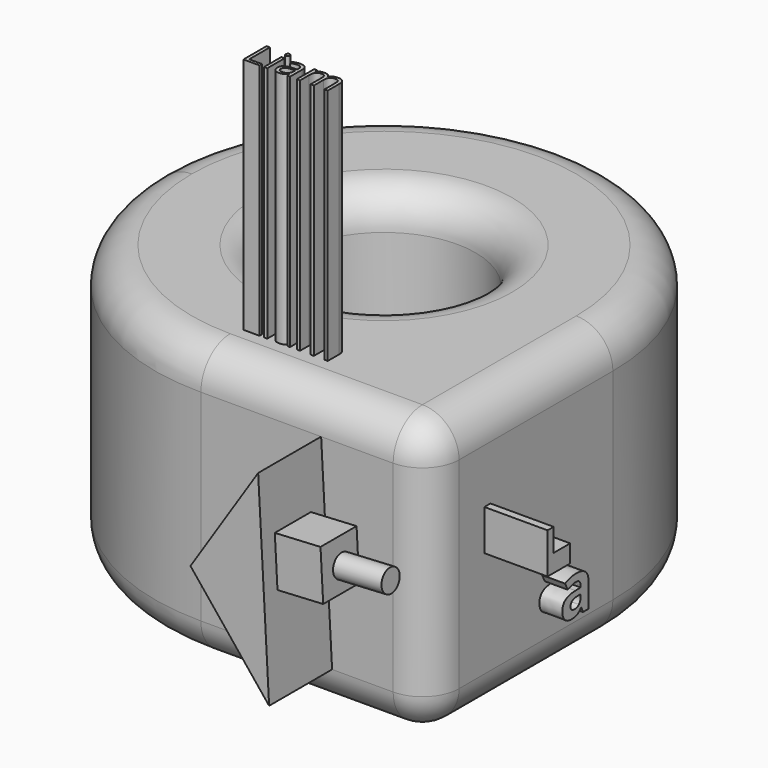
from build123d import *

# Parameters (mm, degrees)
F0_W          = 127
F0_H          = 127
F1_DEPTH      = 76.2
F3_DEPTH      = 84.582
F4_R          = 63.49999
F5_R          = 25.4
F6_DEPTH      = 85.09
F7_R          = 10.16
F9_DEPTH      = 21.844
F10_W         = 12.5058554592
F10_H         = 13.7337893248
F11_DEPTH     = 12.7
F12_R         = 3.150764017
F13_DEPTH     = 13.462
F15_DEPTH     = 17.526
F17_DEPTH     = 6.35
F18_TEXT_SIZE = 11.2532431053
F19_DEPTH     = 66.04


# Not quite as in the source:
# - a fillet or chamfer is up to 0.001 mm smaller than in the source, because OpenCascade refuses the exact size
# - Text() gives the source's letters only with a copy of the font that has no kerning and outlines rounded to 1/6400 em; it was checked with that copy


with BuildPart() as f1:
    # F0 (on Top) → F1 (new body)
    with BuildSketch(Plane.XY):
        Rectangle(F0_W, F0_H)
    extrude(amount=F1_DEPTH)

    # F2 (on face) → F3 (cut)
    with BuildSketch(Plane.XY.offset(76.2)):
        with BuildLine():
            ThreePointArc((1.088e-07, 63.5), (44.9012806438, 44.9012805669), (63.5, 0))
            Line((63.5, 0), (63.5, 63.5))
            Line((63.5, 63.5), (1.088e-07, 63.5))
        make_face()
        with BuildLine():
            ThreePointArc((-63.5, 0), (-44.9012805669, 44.9012806438), (1.088e-07, 63.5))
            Line((1.088e-07, 63.5), (-63.5, 63.5))
            Line((-63.5, 63.5), (-63.5, 0))
        make_face()
    extrude(amount=-F3_DEPTH, mode=Mode.SUBTRACT)

    # F4 (radius 63.5 in the source; OpenCascade refuses exactly that, so slightly less here)
    f4_edges = [f1.edges().sort_by_distance(p)[0] for p in [
        (-63.5, -63.5, 38.1),
    ]]
    fillet(f4_edges, radius=F4_R)

    # F5 (on face) → F6 (cut)
    with BuildSketch(Plane.XY.offset(76.2)):
        Circle(F5_R)
    extrude(amount=-F6_DEPTH, mode=Mode.SUBTRACT)

    # F7
    f7_edges = [f1.edges().sort_by_distance(p)[0] for p in [
        (63.5, -31.75, 0),
        (63.5, 0, 38.1),
        (63.5, -31.75, 76.2),
        (63.5, -63.5, 38.1),
        (31.749995, -63.5, 0),
        (-1e-05, -63.5, 38.1),
        (31.749995, -63.5, 76.2),
        (-25.4, 0, 76.2),
        (25.4, 0, 38.1),
        (-25.4, 0, 0),
    ]]
    fillet(f7_edges, radius=F7_R)

    # F8 (on face) → F9 (join)
    with BuildSketch(Plane.XZ.offset(63.5)):
        Polygon((33.3577431738, 66.04), (14.5826684311, 37.2163690627), (36.4012047648, 10.16), align=None)
    extrude(amount=F9_DEPTH)

    # F10 (on face) → F11 (join)
    with BuildSketch(Plane(origin=(36.8452653483, 0, 2.0067492824), x_dir=(0, 1, 0), z_dir=(0.998520115, 0, 0.0543836367))):
        with Locations((-74.422, 41.0005301237)):
            Rectangle(F10_W, F10_H)
    extrude(amount=F11_DEPTH)

    # F12 (on face) → F13 (join)
    with BuildSketch(Plane(origin=(49.5264708088, 0, 2.6974214682), x_dir=(0, 1, 0), z_dir=(0.998520115, 0, 0.0543836367))):
        with Locations((-73.6612937806, 40.5637623921)):
            Circle(F12_R)
    extrude(amount=F13_DEPTH)

    # F14 (on face) → F15 (join)
    with BuildSketch(Plane.YZ.offset(63.5)):
        Polygon((-42.4495339394, 50.9560592473), (-44.5624440908, 50.9560592473), (-44.5624440908, 39.671652019), (-36.708496511, 39.671652019), (-36.708496511, 44.5811226964), (-42.4495339394, 44.5811226964), align=None)
    extrude(amount=F15_DEPTH)

    # F16 (on face) → F17 (join)
    with BuildSketch(Plane.YZ.offset(63.5)):
        with BuildLine():
            Line((-18.8706061308, 18.0784155527), (-18.3313372545, 16.6938062757))
            Line((-18.3313372545, 16.6938062757), (-16.3928842667, 16.6938062757))
            Line((-16.3928842667, 16.6938062757), (-16.3928842667, 23.4798492165))
            add(Edge.make_bspline(
                [(-17.4859968538, 26.1951408829), (-16.3928842667, 25.3017035284), (-16.3928842667, 23.4798492165)],
                knots=[0, 0, 0, 1, 1, 1], degree=2))
            add(Edge.make_bspline(
                [(-20.6283311709, 27.0885782375), (-18.5791094409, 27.0885782375), (-17.4859968538, 26.1951408829)],
                knots=[0, 0, 0, 1, 1, 1], degree=2))
            add(Edge.make_bspline(
                [(-24.5256419148, 26.1674486974), (-22.7679168747, 27.0885782375), (-20.6283311709, 27.0885782375)],
                knots=[0, 0, 0, 1, 1, 1], degree=2))
            Line((-24.5256419148, 26.1674486974), (-23.6074273416, 24.2902100144))
            add(Edge.make_bspline(
                [(-20.7361849461, 25.0276966399), (-21.9575560768, 25.0276966399), (-23.6074273416, 24.2902100144)],
                knots=[0, 0, 0, 1, 1, 1], degree=2))
            add(Edge.make_bspline(
                [(-19.1504429531, 23.4798492165), (-19.1504429531, 25.0276966399), (-20.7361849461, 25.0276966399)],
                knots=[0, 0, 0, 1, 1, 1], degree=2))
            Line((-19.1504429531, 23.4798492165), (-19.1504429531, 23.033859281))
            Line((-19.1504429531, 23.033859281), (-20.9198278608, 22.9784749099))
            add(Edge.make_bspline(
                [(-24.3390840333, 22.1273045754), (-23.2051619096, 22.8968558367), (-20.9198278608, 22.9784749099)],
                knots=[0, 0, 0, 1, 1, 1], degree=2))
            add(Edge.make_bspline(
                [(-25.473006157, 19.7370317183), (-25.473006157, 21.3577533141), (-24.3390840333, 22.1273045754)],
                knots=[0, 0, 0, 1, 1, 1], degree=2))
            add(Edge.make_bspline(
                [(-24.6305807232, 17.349673828), (-25.473006157, 18.1891842949), (-25.473006157, 19.7370317183)],
                knots=[0, 0, 0, 1, 1, 1], degree=2))
            add(Edge.make_bspline(
                [(-22.3219269392, 16.5101633611), (-23.7881552894, 16.5101633611), (-24.6305807232, 17.349673828)],
                knots=[0, 0, 0, 1, 1, 1], degree=2))
            add(Edge.make_bspline(
                [(-20.3863889183, 16.8526719717), (-21.1297054775, 16.5101633611), (-22.3219269392, 16.5101633611)],
                knots=[0, 0, 0, 1, 1, 1], degree=2))
            add(Edge.make_bspline(
                [(-18.9434803033, 18.0784155527), (-19.643072359, 17.1951805823), (-20.3863889183, 16.8526719717)],
                knots=[0, 0, 0, 1, 1, 1], degree=2))
            Line((-18.9434803033, 18.0784155527), (-18.8706061308, 18.0784155527))
        make_face()
        with BuildLine():
            Line((-20.2260657388, 21.3752431155), (-19.1504429531, 21.4131376852))
            Line((-19.1504429531, 21.4131376852), (-19.1504429531, 20.5736272183))
            add(Edge.make_bspline(
                [(-19.7290638826, 19.0986539674), (-19.1504429531, 19.6554126451), (-19.1504429531, 20.5736272183)],
                knots=[0, 0, 0, 1, 1, 1], degree=2))
            add(Edge.make_bspline(
                [(-21.2754538225, 18.5418952897), (-20.307684812, 18.5418952897), (-19.7290638826, 19.0986539674)],
                knots=[0, 0, 0, 1, 1, 1], degree=2))
            add(Edge.make_bspline(
                [(-22.6221685298, 19.7195419169), (-22.6221685298, 18.5418952897), (-21.2754538225, 18.5418952897)],
                knots=[0, 0, 0, 1, 1, 1], degree=2))
            add(Edge.make_bspline(
                [(-22.0304302493, 20.9394555641), (-22.6221685298, 20.5386476155), (-22.6221685298, 19.7195419169)],
                knots=[0, 0, 0, 1, 1, 1], degree=2))
            add(Edge.make_bspline(
                [(-20.2260657388, 21.3752431155), (-21.4386919688, 21.3402635127), (-22.0304302493, 20.9394555641)],
                knots=[0, 0, 0, 1, 1, 1], degree=2))
        make_face(mode=Mode.SUBTRACT)
    extrude(amount=F17_DEPTH)

    # F18 (on face) → F19 (join)
    with BuildSketch(Plane.XY.offset(76.2)):
        with Locations((0, -50.1369647682)):
            Text('Liam', F18_TEXT_SIZE, font='Open Sans', text_align=(TextAlign.LEFT, TextAlign.BOTTOM))
    extrude(amount=F19_DEPTH)


solid = f1.part
